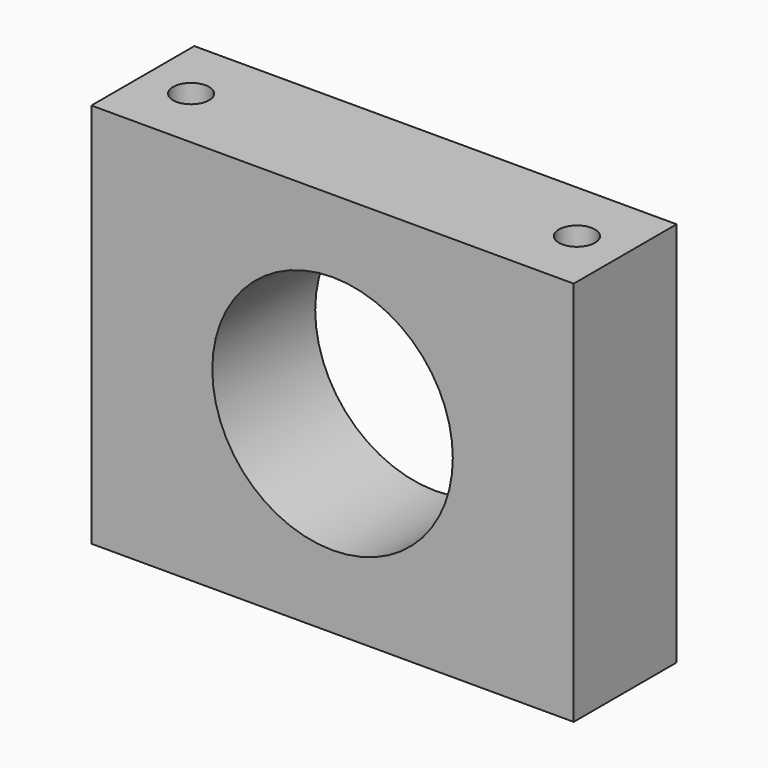
from build123d import *

# Parameters (mm, degrees)
F0_W     = 95.25
F0_H     = 76.2
F0_R     = 23.749
F1_DEPTH = 25.4
F2_R     = 3.5687
F3_DEPTH = 76.201
F4_DEPTH = 76.201


# Not quite as in the source:
# - a feature names something its author has since deleted; it is built from what else it names


with BuildPart() as f1:
    # F0 (on Front) → F1 (new body)
    with BuildSketch(Plane.XZ):
        with Locations((-8.5653835568, 7.273635827)):
            Rectangle(F0_W, F0_H)
        with Locations((-8.5653835568, 7.273635827)):
            Circle(F0_R, mode=Mode.SUBTRACT)
    extrude(amount=F1_DEPTH)

    # F2 (on face) → F3 (cut, through all)
    with BuildSketch(Plane.XY.offset(45.373635827)):
        with Locations((-46.6653835568, -12.7)):
            Circle(F2_R)
    extrude(amount=-F3_DEPTH, mode=Mode.SUBTRACT)

    # F2 (on face) → F4 (cut, through all)
    with BuildSketch(Plane.XY.offset(45.373635827)):
        with Locations((-46.6653835568, -12.7)):
            Circle(F2_R)
        with Locations((29.5346164432, -12.7)):
            Circle(F2_R)
    extrude(amount=-F4_DEPTH, mode=Mode.SUBTRACT)


solid = f1.part
